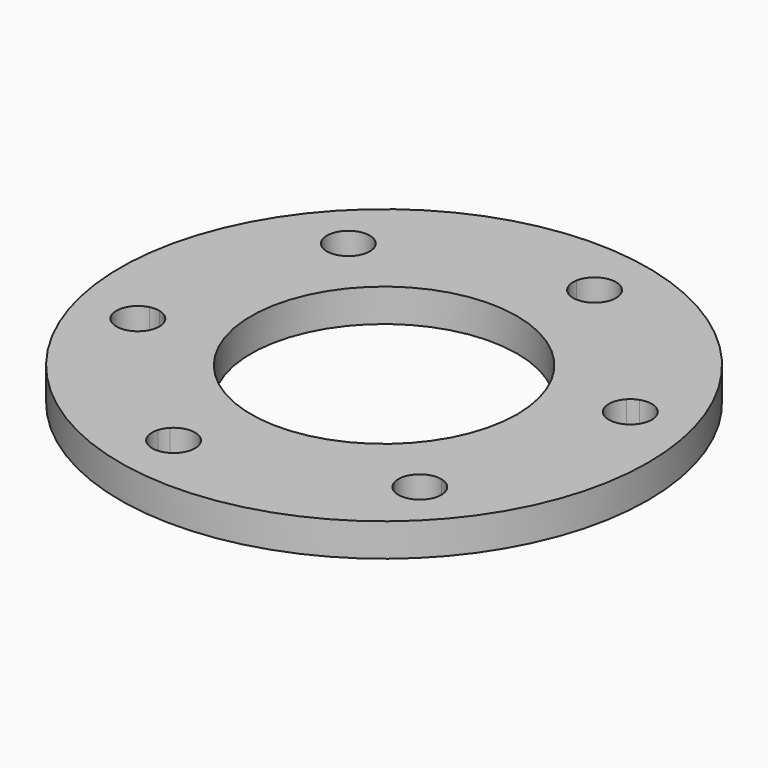
from build123d import *

# Parameters (mm, degrees)
F0_R     = 50.796035682
F1_DEPTH = 6.35
F0_R_2   = 25.5997355282
F2_DEPTH = 6.35


with BuildPart() as f1:
    # F0 (on Top) → F1 (new body)
    with BuildSketch(Plane.XY):
        Circle(F0_R)
        with BuildLine():
            ThreePointArc((39.3271974597, 7.2596428653), (39.8251792413, 3.6449928619), (39.9916350574, 0))
            ThreePointArc((39.9916350574, 0), (37.8457361774, -12.9240522963), (31.638331797, -24.4611290759))
            ThreePointArc((31.638331797, -24.4611290759), (32.6975616463, -25.8682109338), (33.0734716269, -27.5888325992))
            ThreePointArc((33.0734716269, -27.5888325992), (30.4751171589, -31.421463006), (25.9528595707, -30.4266323255))
            ThreePointArc((25.9528595707, -30.4266323255), (11.2745427029, -38.3694613124), (-5.3673629967, -39.6298156572))
            ThreePointArc((-5.3673629967, -39.6298156572), (-10.3899431598, -42.8710411012), (-13.3713628706, -37.6900189645))
            ThreePointArc((-13.3713628706, -37.6900189645), (-27.5888779577, -28.9514194402), (-37.0021800615, -15.1713396))
            ThreePointArc((-37.0021800615, -15.1713396), (-42.3272537393, -12.438997445), (-39.3271186708, -7.2600696702))
            ThreePointArc((-39.3271186708, -7.2600696702), (-38.8660161768, 9.4214468691), (-31.637317072, 24.4624414777))
            ThreePointArc((-31.637317072, 24.4624414777), (-31.9331144569, 30.4341189249), (-25.9541217074, 30.4255557215))
            ThreePointArc((-25.9541217074, 30.4255557215), (-11.2785991848, 38.3682691165), (5.3606272578, 39.6307273459))
            ThreePointArc((5.3606272578, 39.6307273459), (9.8039037737, 42.9758363595), (13.548769251, 38.8638486327))
            ThreePointArc((13.548769251, 38.8638486327), (13.5057955215, 38.2696140057), (13.3777686423, 37.6877457633))
            ThreePointArc((13.3777686423, 37.6877457633), (27.5911811268, 28.9492244903), (37.0020154097, 15.1717411718))
            ThreePointArc((37.0020154097, 15.1717411718), (40.7552771421, 14.6424823027), (42.495179297, 11.2750160335))
            ThreePointArc((42.495179297, 11.2750160335), (41.6078280146, 8.7177063827), (39.3271974597, 7.2596428653))
        make_face(mode=Mode.SUBTRACT)
    extrude(amount=F1_DEPTH)



with BuildPart() as f1b:
    # F0 (on Top) → F1, piece 2 (new body)
    with BuildSketch(Plane.XY):
        with BuildLine():
            Line((29.9194537324, -23.5791233665), (37.3940186124, 7.2624677043))
            ThreePointArc((37.3940186124, 7.2624677043), (34.4052772179, 10.1109124169), (35.3777320032, 14.1234607462))
            Line((35.3777320032, 14.1234607462), (12.4084521668, 36.0145229256))
            ThreePointArc((12.4084521668, 36.0145229256), (8.4460308303, 34.8500592639), (5.4563650491, 37.6993849709))
            Line((5.4563650491, 37.6993849709), (-24.9908830503, 28.7516454448))
            ThreePointArc((-24.9908830503, 28.7516454448), (-24.8656043881, 28.1762274896), (-24.8235590671, 27.5888325992))
            ThreePointArc((-24.8235590671, 27.5888325992), (-26.3979468028, 24.3473427918), (-29.9190635285, 23.5807334278))
            Line((-29.9190635285, 23.5807334278), (-37.3941206986, -7.2628889331))
            ThreePointArc((-37.3941206986, -7.2628889331), (-35.1217260633, -8.7227134695), (-34.2382009209, -11.2750160335))
            ThreePointArc((-34.2382009209, -11.2750160335), (-34.5337408719, -12.8088983718), (-35.3780457549, -14.1231617225))
            Line((-35.3780457549, -14.1231617225), (-12.4035384742, -36.019205961))
            ThreePointArc((-12.4035384742, -36.019205961), (-8.4476296116, -34.8566561642), (-5.4628775231, -37.7012988359))
            Line((-5.4628775231, -37.7012988359), (24.9892935944, -28.752112549))
            ThreePointArc((24.9892935944, -28.752112549), (25.9610603149, -24.7424033164), (29.9194537324, -23.5791233665))
        make_face()
        Circle(F0_R_2, mode=Mode.SUBTRACT)
    extrude(amount=F1_DEPTH)


with BuildPart() as f1_1:
    add(f1.part)

    add(f1b.part)  # F2 merges F1b
    # F0 (on Top) → F2 (join)
    with BuildSketch(Plane.XY):
        with BuildLine():
            ThreePointArc((31.638331797, -24.4611290759), (37.8457361774, -12.9240522963), (39.9916350574, 0))
            ThreePointArc((39.9916350574, 0), (39.8251792413, 3.6449928619), (39.3271974597, 7.2596428653))
            ThreePointArc((39.3271974597, 7.2596428653), (38.3604403722, 7.146314542), (37.3940186124, 7.2624677043))
            Line((37.3940186124, 7.2624677043), (29.9194537324, -23.5791233665))
            ThreePointArc((29.9194537324, -23.5791233665), (30.8312469464, -23.9180968879), (31.638331797, -24.4611290759))
        make_face()
        with BuildLine():
            ThreePointArc((35.3777320032, 14.1234607462), (36.1276546961, 14.7440077063), (37.0020154097, 15.1717411718))
            ThreePointArc((37.0020154097, 15.1717411718), (27.5911811268, 28.9492244903), (13.3777686423, 37.6877457633))
            ThreePointArc((13.3777686423, 37.6877457633), (12.9924184393, 36.7936041028), (12.4084521668, 36.0145229256))
            Line((12.4084521668, 36.0145229256), (35.3777320032, 14.1234607462))
        make_face()
        with BuildLine():
            ThreePointArc((-5.3673629967, -39.6298156572), (11.2745427029, -38.3694613124), (25.9528595707, -30.4266323255))
            ThreePointArc((25.9528595707, -30.4266323255), (25.3716802728, -29.6465678813), (24.9892935944, -28.752112549))
            Line((24.9892935944, -28.752112549), (-5.4628775231, -37.7012988359))
            ThreePointArc((-5.4628775231, -37.7012988359), (-5.3376272012, -38.2765866213), (-5.2955913916, -38.8638486327))
            ThreePointArc((-5.2955913916, -38.8638486327), (-5.3135735047, -39.2485097322), (-5.3673629967, -39.6298156572))
        make_face()
        with BuildLine():
            ThreePointArc((5.4563650491, 37.6993849709), (5.2938683757, 38.6593739913), (5.3606272578, 39.6307273459))
            ThreePointArc((5.3606272578, 39.6307273459), (-11.2785991848, 38.3682691165), (-25.9541217074, 30.4255557215))
            ThreePointArc((-25.9541217074, 30.4255557215), (-25.3731377903, 29.6457791632), (-24.9908830503, 28.7516454448))
            Line((-24.9908830503, 28.7516454448), (5.4563650491, 37.6993849709))
        make_face()
        with BuildLine():
            ThreePointArc((-37.0021800615, -15.1713396), (-27.5888779577, -28.9514194402), (-13.3713628706, -37.6900189645))
            ThreePointArc((-13.3713628706, -37.6900189645), (-12.9866339101, -36.7971602183), (-12.4035384742, -36.019205961))
            Line((-12.4035384742, -36.019205961), (-35.3780457549, -14.1231617225))
            ThreePointArc((-35.3780457549, -14.1231617225), (-36.1278992542, -14.7436496905), (-37.0021800615, -15.1713396))
        make_face()
        with BuildLine():
            ThreePointArc((-29.9190635285, 23.5807334278), (-30.8305291615, 23.9195906141), (-31.637317072, 24.4624414777))
            ThreePointArc((-31.637317072, 24.4624414777), (-38.8660161768, 9.4214468691), (-39.3271186708, -7.2600696702))
            ThreePointArc((-39.3271186708, -7.2600696702), (-38.3604523499, -7.1467479477), (-37.3941206986, -7.2628889331))
            Line((-37.3941206986, -7.2628889331), (-29.9190635285, 23.5807334278))
        make_face()
    extrude(amount=F2_DEPTH)


solid = f1_1.part
